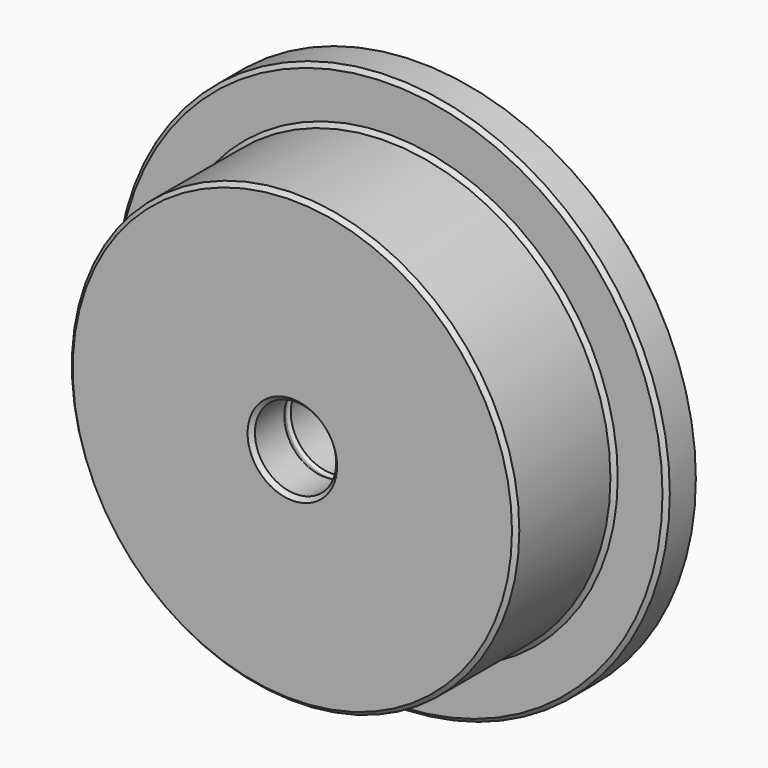
from build123d import *

# Parameters (mm, degrees)
F0_R     = 34
F1_DEPTH = 5
F2_R     = 27.5
F3_DEPTH = 15
F4_R     = 5
F5_DEPTH = 30
F6_SIZE  = 0.5
F8_R     = 5.25
F9_DEPTH = 1


# Not quite as in the source:
# - a fillet or chamfer that OpenCascade refuses, or shapes differently, is made with other operations: its cross-section is extruded or revolved along the edge and cut away or added


with BuildPart() as f1:
    # F0 (on Front) → F1 (new body)
    with BuildSketch(Plane.XZ):
        Circle(F0_R)
    extrude(amount=F1_DEPTH)

    # F2 (on face) → F3 (join)
    with BuildSketch(Plane.XZ.offset(5)):
        Circle(F2_R)
    extrude(amount=F3_DEPTH)

    # F4 (on face) → F5 (cut)
    with BuildSketch(Plane.XZ.offset(20)):
        Circle(F4_R)
    extrude(amount=-F5_DEPTH, mode=Mode.SUBTRACT)

    # F6
    f6_edges = [f1.edges().sort_by_distance(p)[0] for p in [
        (-34, 0, 0),
        (-27.5, -20, 0),
        (-34, -5, 0),
        (-27.5, -5, 0),
        (-5, -20, 0),
        (-5, 0, 0),
    ]]
    chamfer(f6_edges, length=F6_SIZE)

    # F8 (on offset) → F9 (cut)
    with BuildSketch(Plane.XZ.offset(15)):
        Circle(F8_R)
    extrude(amount=-F9_DEPTH, mode=Mode.SUBTRACT)

    # F10: fillet of radius 0.5 on 3 edges, made by hand

    # F10_s1 → F10_t2 (revolve)
    with BuildSketch(Plane.XY):
        with BuildLine():
            ThreePointArc((5.25, -14.5669872981), (5.1830127019, -14.8169872981), (5, -15))
            Line((5, -15), (5.25, -15))
            Line((5.25, -15), (5.25, -14.5669872981))
        make_face()
    revolve(axis=Axis((0, -15, 0), (0, -1, 0)))

    # F10_s3 → F10_t4 (revolve)
    with BuildSketch(Plane.XY):
        with BuildLine():
            ThreePointArc((5, -14), (5.1830127019, -14.1830127019), (5.25, -14.4330127019))
            Line((5.25, -14.4330127019), (5.25, -14))
            Line((5.25, -14), (5, -14))
        make_face()
    revolve(axis=Axis((0, -14, 0), (0, -1, 0)))


solid = f1.part
